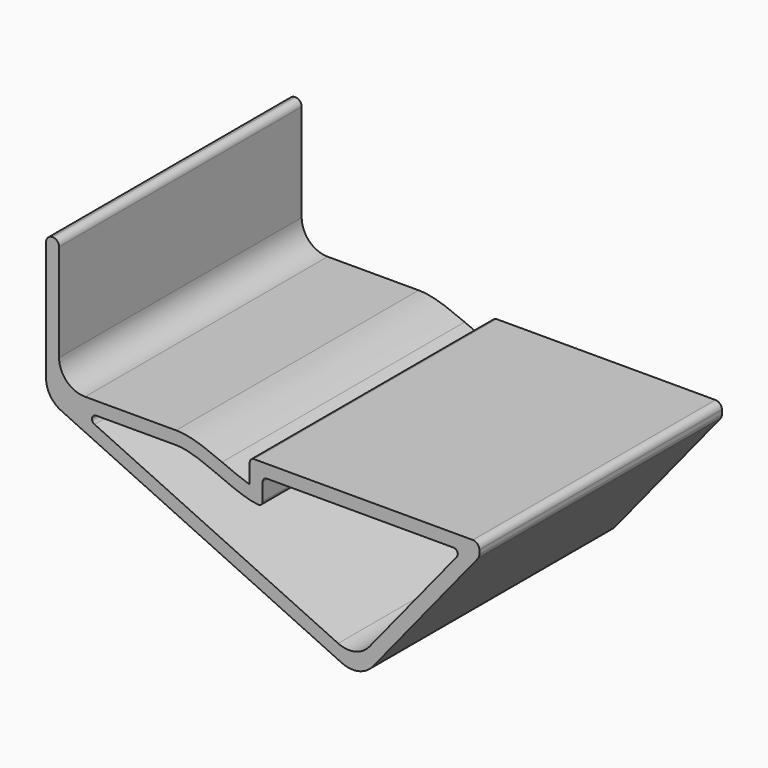
from build123d import *

# Parameters (mm, degrees)
F0_W         = 1.5
F0_H         = 15
F0_H_2       = 1.5
F1_DEPTH     = 35
F2_R         = 3
F3_R         = 0.5
F4_R         = 0.74999
F5_TEXT_SIZE = 7.8123211902
F6_DEPTH     = 0.4


# Not quite as in the source:
# - a fillet or chamfer is up to 0.001 mm smaller than in the source, because OpenCascade refuses the exact size
# - ends of sketch curves that miss each other by under 0.0002 mm in the source are joined
# - Text() gives the source's letters only with a copy of the font that has no kerning and outlines rounded to 1/6400 em; it was checked with that copy


with BuildPart() as f1:
    # F0 (on Front) → F1 (new body)
    with BuildSketch(Plane.XZ):
        with Locations((0.75, 9)):
            Rectangle(F0_W, F0_H)
        with BuildLine():
            Line((1.5, 1.5), (0, 1.5))
            Line((0, 1.5), (0, 0))
            Line((0, 0), (3.5493023747, 0))
            Line((3.5493023747, 0), (15, 0))
            Line((15, 0), (20.3076726165, 0))
            add(Edge.make_bspline(
                [(20.3076726165, 0), (19.9613391426, 0.1480763703), (19.1624921639, 0.4865686334), (17.8864112021, 0.9748848409), (16.4769611274, 1.3772161031), (15.5, 1.5), (15, 1.5)],
                knots=[0.5268596167, 0.5268596167, 0.5268596167, 0.5268596167, 0.625, 0.75, 0.875, 1, 1, 1, 1], degree=3))
            Line((15, 1.5), (1.5, 1.5))
        make_face()
        with BuildLine():
            add(Edge.make_bspline(
                [(23.5000271172, -1.2432669014), (23.3597225948, -1.2025116169), (22.8440957766, -1.0410149339), (21.8859439585, -0.6761057841), (20.9362434779, -0.2693177997), (20.4024591259, -0.0405263808), (20.3076726165, 0)],
                knots=[0.2014712136, 0.2014712136, 0.2014712136, 0.2014712136, 0.25, 0.375, 0.5, 0.5268596167, 0.5268596167, 0.5268596167, 0.5268596167], degree=3))
            Line((20.3076726165, 0), (15, 0))
            add(Edge.make_bspline(
                [(25, -3), (22, -3), (18, 0), (15, 0)],
                knots=[0, 0, 0, 0, 10.4403065089, 10.4403065089, 10.4403065089, 10.4403065089], degree=3))
            Line((25, -3), (25, 0))
            Line((25, 0), (23.5, 0))
            Line((23.5, 0), (23.5000271172, -1.2432669014))
        make_face()
        with Locations((24.25, 0.75)):
            Rectangle(F0_W, F0_H_2)
        Polygon((48.0665893009, 0), (50, 0), (50, 1.5), (25, 1.5), (25, 0), align=None)
        Polygon((36.8862388741, -15.5452687891), (36.2523114815, -16.9047304696), (50, 0), (48.0665893009, 0), (35.8263934139, -15.0510547345), align=None)
        Polygon((3.5493023747, 0), (0, 0), (36.2523114815, -16.9047304696), (36.8862388741, -15.5452687891), (35.8263934139, -15.0510547345), align=None)
    extrude(amount=F1_DEPTH)

    # F2
    f2_edges = [f1.edges().sort_by_distance(p)[0] for p in [
        (1.5, -17.5, 1.5),
        (0, -17.5, 0),
        (36.252311, -17.5, -16.90473),
        (35.826393, -17.5, -15.051055),
    ]]
    fillet(f2_edges, radius=F2_R)

    # F3
    f3_edges = [f1.edges().sort_by_distance(p)[0] for p in [
        (48.066589, -17.5, 0),
        (3.549302, -17.5, 0),
        (15, -17.5, 0),
        (23.5, -17.5, 1.5),
        (25, -17.5, 0),
        (25, -17.5, -3),
    ]]
    fillet(f3_edges, radius=F3_R)

    # F4 (radius 0.75 in the source; OpenCascade refuses exactly that, so slightly less here)
    f4_edges = [f1.edges().sort_by_distance(p)[0] for p in [
        (50, -17.5, 0),
        (50, -17.5, 1.5),
        (1.5, -17.5, 16.5),
        (0, -17.5, 16.5),
    ]]
    fillet(f4_edges, radius=F4_R)

    # F5 (on face) → F6 (cut)
    with BuildSketch(Plane(origin=(0, 0, 0), x_dir=(0.906307787, 0, -0.4226182617), z_dir=(-0.4226182617, 0, -0.906307787))):
        with Locations((3.7861953129, 14.6875643715)):
            Text('AIRSTER', F5_TEXT_SIZE, font='Open Sans', font_style=FontStyle.BOLD, text_align=(TextAlign.LEFT, TextAlign.BOTTOM))
    extrude(amount=-F6_DEPTH, mode=Mode.SUBTRACT)


solid = f1.part
